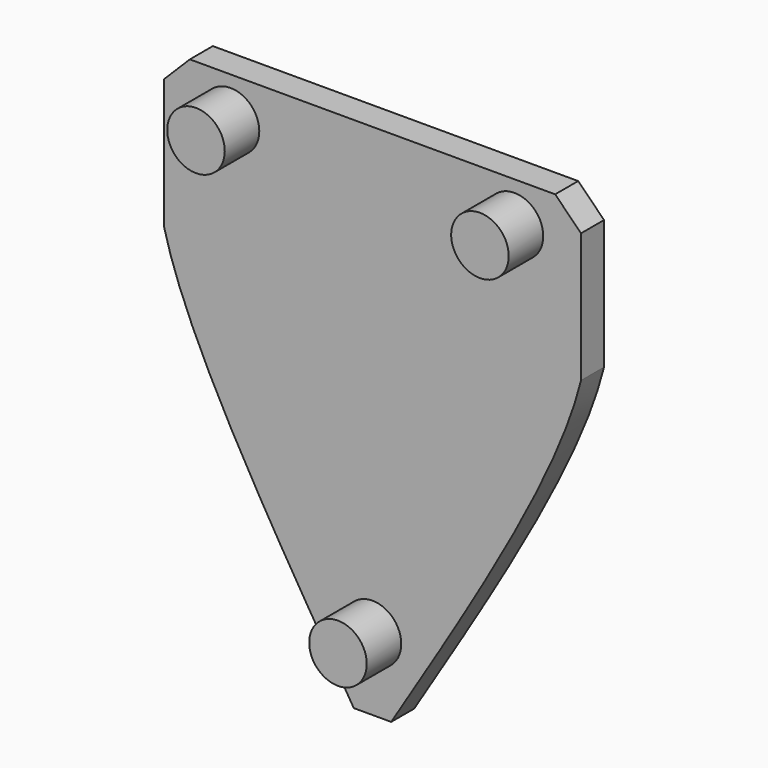
from build123d import *

# Parameters (mm, degrees)
F1_DEPTH = 20
F2_R     = 20
F3_DEPTH = 30


with BuildPart() as f1:
    # F0 (on Front) → F1 (new body)
    with BuildSketch(Plane.XZ):
        with BuildLine():
            add(Edge.make_bspline(
                [(0, 0), (15.8393937026, -64.3749522899), (73.9196968513, -158.1874761449), (132, -252)],
                knots=[0.3599862205, 0.3599862205, 0.3599862205, 0.3599862205, 1, 1, 1, 1], degree=3))
            Line((132, -252), (158, -252))
            add(Edge.make_bspline(
                [(290, 0), (274.1606062974, -64.3749522899), (216.0803031487, -158.1874761449), (158, -252)],
                knots=[0.3599862205, 0.3599862205, 0.3599862205, 0.3599862205, 1, 1, 1, 1], degree=3))
            Line((290, 0), (290, 90))
            Line((290, 90), (272, 108))
            Line((272, 108), (18, 108))
            Line((18, 108), (0, 90))
            Line((0, 90), (0, 0))
        make_face()
    extrude(amount=F1_DEPTH)

    # F2 (on face) → F3 (join)
    with BuildSketch(Plane.XZ.offset(20)):
        with Locations((46.2842712475, 79.7157287525)):
            Circle(F2_R)
        with Locations((243.7157287525, 79.7157287525)):
            Circle(F2_R)
        with Locations((145, -202)):
            Circle(F2_R)
    extrude(amount=F3_DEPTH)


solid = f1.part
